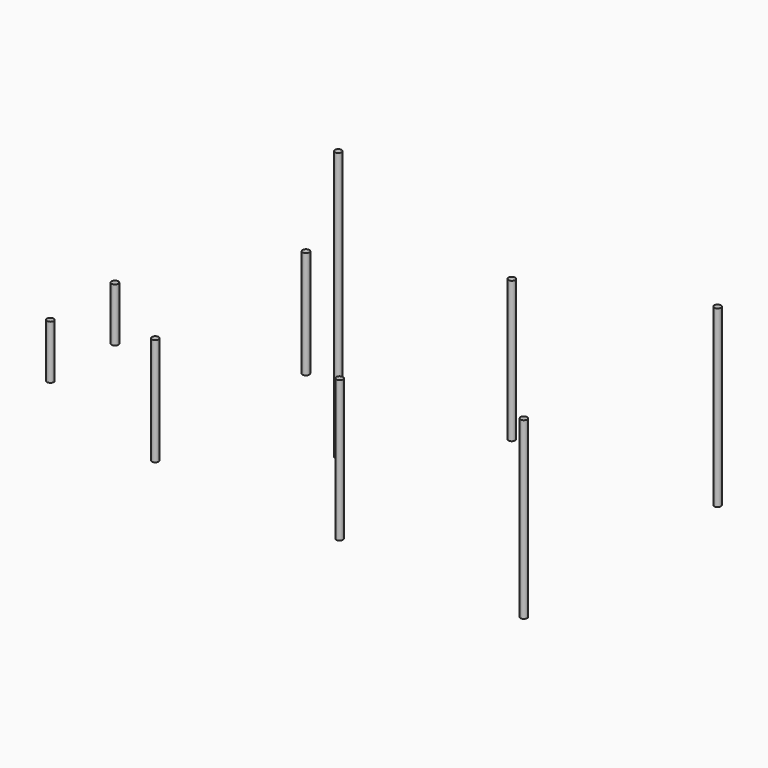
from build123d import *

# Parameters (mm, degrees)
F1_R     = 76.2
F2_DEPTH = 1219.2
F3_DEPTH = 2438.4
F4_DEPTH = 6096
F5_DEPTH = 3200.4
F6_DEPTH = 3962.4


# Not quite as in the source:
# - the program builds the solid bodies; features that only make, move or delete a surface that nothing else refers to are left out


with BuildPart() as f2:
    # F1 (on Top) → F2 (new body)
    with BuildSketch(Plane.XY):
        with Locations((-6553.2, 914.4)):
            Circle(F1_R)
    extrude(amount=F2_DEPTH)


with BuildPart() as f2b:
    # F1 (on Top) → F2, piece 2 (new body)
    with BuildSketch(Plane.XY):
        with Locations((-6553.2, -914.4)):
            Circle(F1_R)
    extrude(amount=F2_DEPTH)


with BuildPart() as f3:
    # F1 (on Top) → F3 (new body)
    with BuildSketch(Plane.XY):
        with Locations((-3200.4, 2133.6)):
            Circle(F1_R)
    extrude(amount=F3_DEPTH)


with BuildPart() as f3b:
    # F1 (on Top) → F3, piece 2 (new body)
    with BuildSketch(Plane.XY):
        with Locations((-3200.4, -2133.6)):
            Circle(F1_R)
    extrude(amount=F3_DEPTH)


with BuildPart() as f4:
    # F1 (on Top) → F4 (new body)
    with BuildSketch(Plane.XY):
        with Locations((-762, 0)):
            Circle(F1_R)
    extrude(amount=F4_DEPTH)


with BuildPart() as f5:
    # F1 (on Top) → F5 (new body)
    with BuildSketch(Plane.XY):
        with Locations((1219.2, 2438.4)):
            Circle(F1_R)
    extrude(amount=F5_DEPTH)


with BuildPart() as f5b:
    # F1 (on Top) → F5, piece 2 (new body)
    with BuildSketch(Plane.XY):
        with Locations((1219.2, -2438.4)):
            Circle(F1_R)
    extrude(amount=F5_DEPTH)


with BuildPart() as f6:
    # F1 (on Top) → F6 (new body)
    with BuildSketch(Plane.XY):
        with Locations((5638.8, 2743.2)):
            Circle(F1_R)
    extrude(amount=F6_DEPTH)


with BuildPart() as f6b:
    # F1 (on Top) → F6, piece 2 (new body)
    with BuildSketch(Plane.XY):
        with Locations((5638.8, -2743.2)):
            Circle(F1_R)
    extrude(amount=F6_DEPTH)


solid = Compound([f2.part, f2b.part, f3.part, f3b.part, f4.part, f5.part, f5b.part, f6.part, f6b.part])
